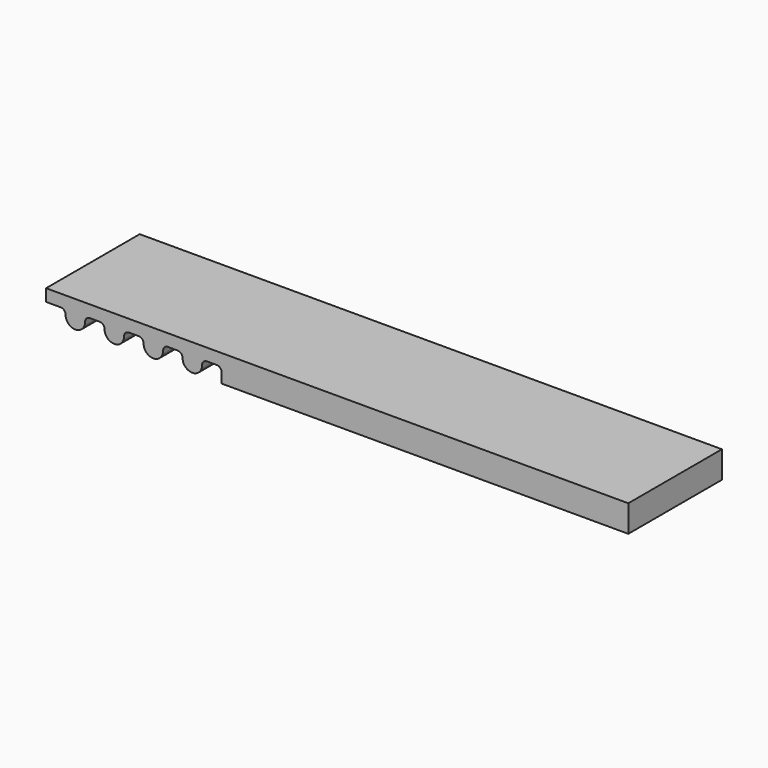
from build123d import *

# Parameters (mm, degrees)
F0_W     = 29.8571444048
F0_H     = 6
F1_DEPTH = 1.38
F2_W     = 1
F2_H     = 6
F3_DEPTH = 0.76
F4_R     = 0.49999
F5_R     = 0.25


# Not quite as in the source:
# - a fillet or chamfer is up to 0.001 mm smaller than in the source, because OpenCascade refuses the exact size


with BuildPart() as f1:
    # F0 (on Top) → F1 (new body)
    with BuildSketch(Plane.XY):
        with Locations((2.9934216291, 0)):
            Rectangle(F0_W, F0_H)
    extrude(amount=F1_DEPTH)

    # F2 (on face) → F3 (cut)
    with BuildSketch(Plane(origin=(0, 0, 0), x_dir=(1, 0, 0), z_dir=(0, 0, -1))):
        with Locations((-11.4351505733, 0)):
            Rectangle(F2_W, F2_H)
        with Locations((-9.4351505733, 0)):
            Rectangle(F2_W, F2_H)
        with Locations((-7.4351505733, 0)):
            Rectangle(F2_W, F2_H)
        with Locations((-5.4351505733, 0)):
            Rectangle(F2_W, F2_H)
        with Locations((-3.4351505733, 0)):
            Rectangle(F2_W, F2_H)
    extrude(amount=-F3_DEPTH, mode=Mode.SUBTRACT)

    # F4 (radius 0.5 in the source; OpenCascade refuses exactly that, so slightly less here)
    f4_edges = [f1.edges().sort_by_distance(p)[0] for p in [
        (-10.935151, 0, 0),
        (-9.935151, 0, 0),
        (-8.935151, 0, 0),
        (-7.935151, 0, 0),
        (-6.935151, 0, 0),
        (-5.935151, 0, 0),
        (-4.935151, 0, 0),
        (-3.935151, 0, 0),
    ]]
    fillet(f4_edges, radius=F4_R)

    # F5
    f5_edges = [f1.edges().sort_by_distance(p)[0] for p in [
        (-10.935151, 0, 0.76),
        (-9.935151, 0, 0.76),
        (-8.935151, 0, 0.76),
        (-6.935151, 0, 0.76),
        (-4.935151, 0, 0.76),
        (-2.935151, 0, 0.76),
        (-3.935151, 0, 0.76),
        (-5.935151, 0, 0.76),
        (-7.935151, 0, 0.76),
    ]]
    fillet(f5_edges, radius=F5_R)


solid = f1.part
